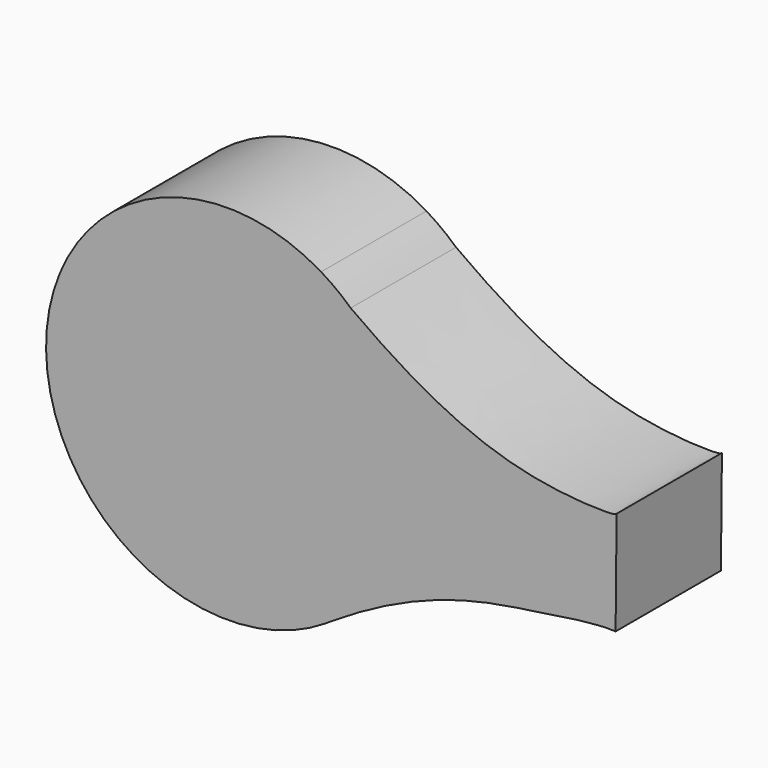
from build123d import *

# Parameters (mm, degrees)
F1_DEPTH = 25.4


with BuildPart() as f1:
    # F0 (on Front) → F1 (new body)
    with BuildSketch(Plane.XZ):
        with BuildLine():
            add(Edge.make_bspline(
                [(-18.2338618332, 35.049978312), (-16.2634742331, 33.5219960414), (-14.3632449685, 32.0948882514), (-12.5260129681, 30.7620231507)],
                knots=[0, 0, 0, 0, 0.065741729, 0.065741729, 0.065741729, 0.065741729], degree=3))
            ThreePointArc((-18.2338618332, 35.049978312), (-71.2893804123, 4.6016135845), (-17.4403864611, -24.4203921477))
            add(Edge.make_bspline(
                [(-17.4403864611, -24.4203921477), (-17.179402441, -24.2472786453), (-16.9196286438, -24.0762946974), (-16.6610557268, -23.9074107575)],
                knots=[0, 0, 0, 0, 0.0086559059, 0.0086559059, 0.0086559059, 0.0086559059], degree=3))
            ThreePointArc((-16.6610557268, -23.9074107575), (-5.3724339888, -11.3311344475), (-1.2924953236, 5.0685547891))
            ThreePointArc((-1.2924953236, 5.0685547891), (-4.2236094492, 19.0894876674), (-12.5260129681, 30.7620231507))
        make_face()
        with BuildLine():
            ThreePointArc((-12.5260129681, 30.7620231507), (-15.2703232487, 33.0519120082), (-18.2338618332, 35.049978312))
            add(Edge.make_bspline(
                [(-18.2338618332, 35.049978312), (-16.2634742331, 33.5219960414), (-14.3632449685, 32.0948882514), (-12.5260129681, 30.7620231507)],
                knots=[0, 0, 0, 0, 0.065741729, 0.065741729, 0.065741729, 0.065741729], degree=3))
        make_face()
        with BuildLine():
            add(Edge.make_bspline(
                [(-17.4403864611, -24.4203921477), (-17.179402441, -24.2472786453), (-16.9196286438, -24.0762946974), (-16.6610557268, -23.9074107575)],
                knots=[0, 0, 0, 0, 0.0086559059, 0.0086559059, 0.0086559059, 0.0086559059], degree=3))
            ThreePointArc((-17.4403864611, -24.4203921477), (-17.0490116738, -24.1664984351), (-16.6610557268, -23.9074107575))
        make_face()
        with BuildLine():
            add(Edge.make_bspline(
                [(-12.5260129681, 30.7620231507), (2.638402042, 19.7606256484), (20.1903372376, 12.3655817594), (38.1732838608, 11.9589753306), (38.6908322584, 12.4428219154), (38.7721241334, 12.5086976901)],
                knots=[0.065741729, 0.065741729, 0.065741729, 0.065741729, 0.6083704565, 0.9417253051, 1, 1, 1, 1], degree=3))
            ThreePointArc((-12.5260129681, 30.7620231507), (-4.2236094492, 19.0894876674), (-1.2924953236, 5.0685547891))
            ThreePointArc((-1.2924953236, 5.0685547891), (-5.3724339888, -11.3311344475), (-16.6610557268, -23.9074107575))
            add(Edge.make_bspline(
                [(-16.6610557268, -23.9074107575), (2.0260763524, -11.7021244239), (14.4410223527, -10.4651605814), (24.1103417725, -9.0437679707)],
                knots=[0.0086559059, 0.0086559059, 0.0086559059, 0.0086559059, 0.6342204815, 0.6342204815, 0.6342204815, 0.6342204815], degree=3))
            add(Edge.make_bspline(
                [(24.1103417725, -9.0437679707), (29.6806384765, -8.2249328253), (34.3397507009, -7.3448917488), (38.5815591641, -7.5473355981)],
                knots=[0.6342204815, 0.6342204815, 0.6342204815, 0.6342204815, 0.9945954099, 0.9945954099, 0.9945954099, 0.9945954099], degree=3))
            add(Edge.make_bspline(
                [(38.5815591641, -7.5473355981), (38.6450808205, -0.6026015768), (38.708602477, 5.5213805001), (38.7721241334, 12.5086976901)],
                knots=[0.5076766633, 0.5076766633, 0.5076766633, 0.5076766633, 20.5853675478, 20.5853675478, 20.5853675478, 20.5853675478], degree=3))
        make_face()
    extrude(amount=F1_DEPTH)


solid = f1.part
